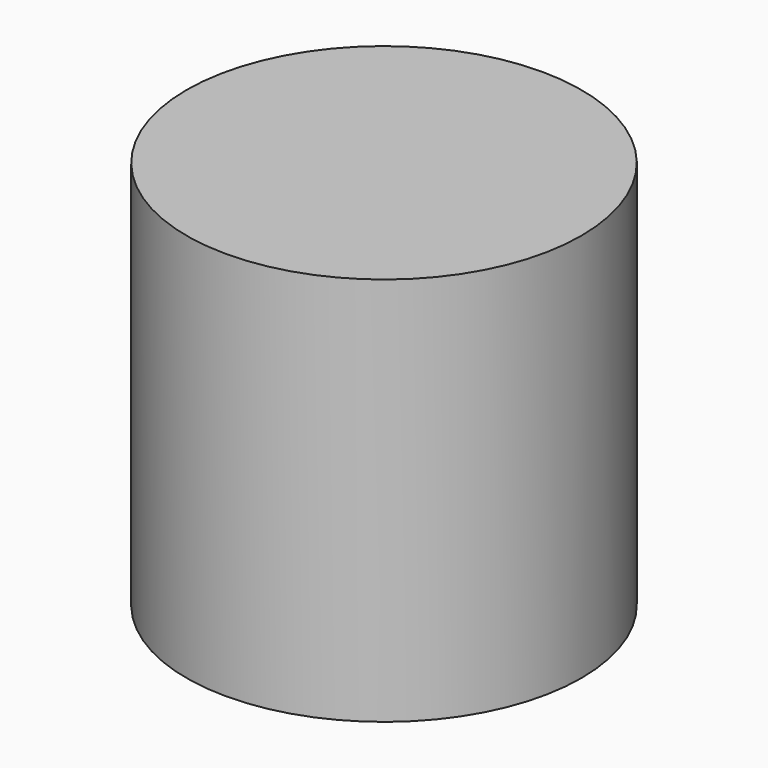
from build123d import *

# Parameters (mm, degrees)
F0_R     = 30.8976987805
F1_DEPTH = 60.96


# Not quite as in the source:
# - the program builds the solid bodies; features that only make, move or delete a surface that nothing else refers to are left out


with BuildPart() as f1:
    # F0 (on Top) → F1 (new body)
    with BuildSketch(Plane.XY):
        Circle(F0_R)
    extrude(amount=F1_DEPTH)


solid = f1.part
